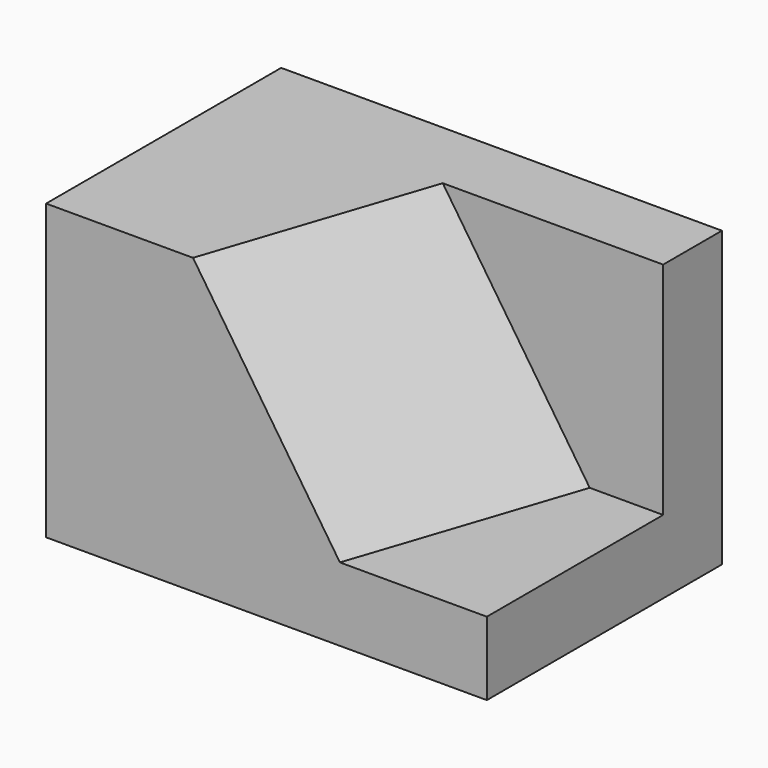
from build123d import *

# Parameters (mm, degrees)
F0_W     = 60
F0_H     = 40
F1_DEPTH = 10


with BuildPart() as f1:
    # F0 (on Top) → F1 (new body)
    with BuildSketch(Plane.XY):
        with Locations((30, 20)):
            Rectangle(F0_W, F0_H)
    extrude(amount=F1_DEPTH)

    # F3 (on offset) → F5 section 0
    with BuildSketch(Plane.XY.offset(40)):
        Polygon((0, 40), (0, 0), (20, 0), (30, 30), (50, 30), (60, 30), (60, 40), align=None)
    # F4 (on face) → F5 section 1
    with BuildSketch(Plane.XY.offset(10)):
        Polygon((50, 30), (60, 30), (60, 40), (0, 40), (0, 0), (40, 0), align=None)
    loft()


solid = f1.part
